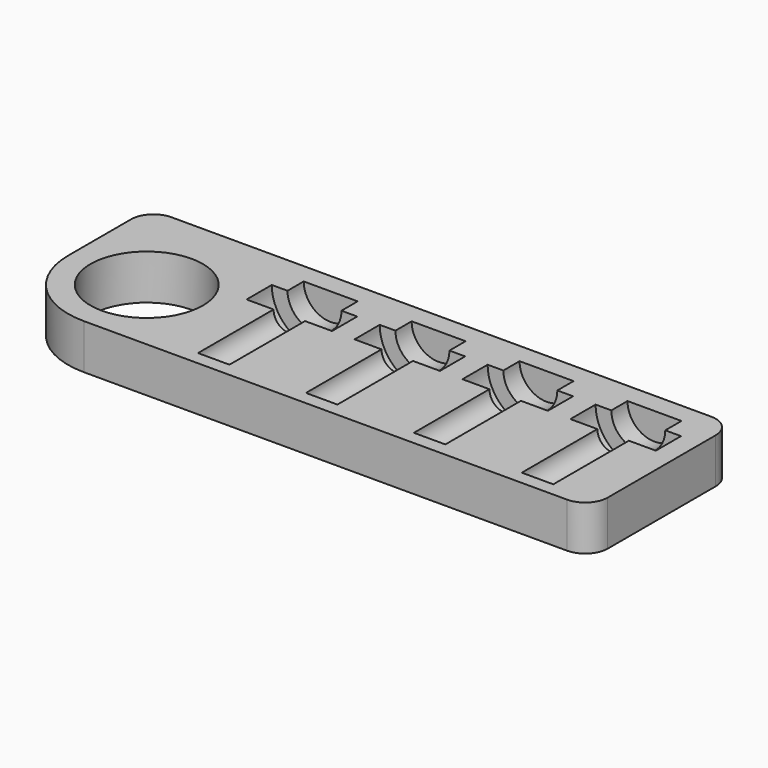
from build123d import *

# Parameters (mm, degrees)
F0_R         = 12.5
F1_DEPTH     = 10
F7_TEXT_SIZE = 5.5555555556
F8_DEPTH     = 1


# Not quite as in the source:
# - Text() gives the source's letters only with a copy of the font that has no kerning and outlines rounded to 1/6400 em; it was checked with that copy


with BuildPart() as f1:
    # F0 (on Top) → F1 (new body)
    with BuildSketch(Plane.XY):
        with BuildLine():
            ThreePointArc((0, 17.5), (5.1256313292, 5.1256313292), (17.5, 0))
            Line((17.5, 0), (125, 0))
            ThreePointArc((125, 0), (128.5355339059, 1.4644660941), (130, 5))
            Line((130, 5), (130, 35))
            ThreePointArc((130, 35), (128.5355339059, 38.5355339059), (125, 40))
            Line((125, 40), (5, 40))
            ThreePointArc((5, 40), (1.4644660941, 38.5355339059), (0, 35))
            Line((0, 35), (0, 17.5))
        make_face()
        with Locations((17.5, 17.5)):
            Circle(F0_R, mode=Mode.SUBTRACT)
    extrude(amount=F1_DEPTH)

    # F2 (on face) → F3 (revolve, cut)
    with BuildSketch(Plane.XY.offset(10)):
        Polygon((44, 24), (44, 3), (47.5, 3), (47.5, 24), (53.5, 24), (53.5, 31), (50, 31), (50, 35.5), (44, 35.5), (44, 31), align=None)
    revolve(axis=Axis((44, 13.5, 10), (0, 1, 0)), mode=Mode.SUBTRACT)

    # F2 (on face) → F4 (revolve, cut)
    with BuildSketch(Plane.XY.offset(10)):
        Polygon((68, 24), (68, 3), (71.5, 3), (71.5, 24), (77.5, 24), (77.5, 31), (74, 31), (74, 35.5), (68, 35.5), (68, 31), align=None)
    revolve(axis=Axis((68, 13.5, 10), (0, 1, 0)), mode=Mode.SUBTRACT)

    # F2 (on face) → F5 (revolve, cut)
    with BuildSketch(Plane.XY.offset(10)):
        Polygon((92, 24), (92, 3), (95.5, 3), (95.5, 24), (101.5, 24), (101.5, 31), (98, 31), (98, 35.5), (92, 35.5), (92, 31), align=None)
    revolve(axis=Axis((92, 13.5, 10), (0, 1, 0)), mode=Mode.SUBTRACT)

    # F2 (on face) → F6 (revolve, cut)
    with BuildSketch(Plane.XY.offset(10)):
        Polygon((116, 24), (116, 3), (119.5, 3), (119.5, 24), (125.5, 24), (125.5, 31), (122, 31), (122, 35.5), (116, 35.5), (116, 31), align=None)
    revolve(axis=Axis((116, 13.5, 10), (0, 1, 0)), mode=Mode.SUBTRACT)

    # F7 (on face) → F8 (cut)
    with BuildSketch(Plane(origin=(0, 0, 0), x_dir=(1, 0, 0), z_dir=(0, 0, -1))):
        with Locations((30, -9)):
            Text('960', F7_TEXT_SIZE, font='Open Sans', text_align=(TextAlign.LEFT, TextAlign.BOTTOM))
    extrude(amount=-F8_DEPTH, mode=Mode.SUBTRACT)


solid = f1.part
